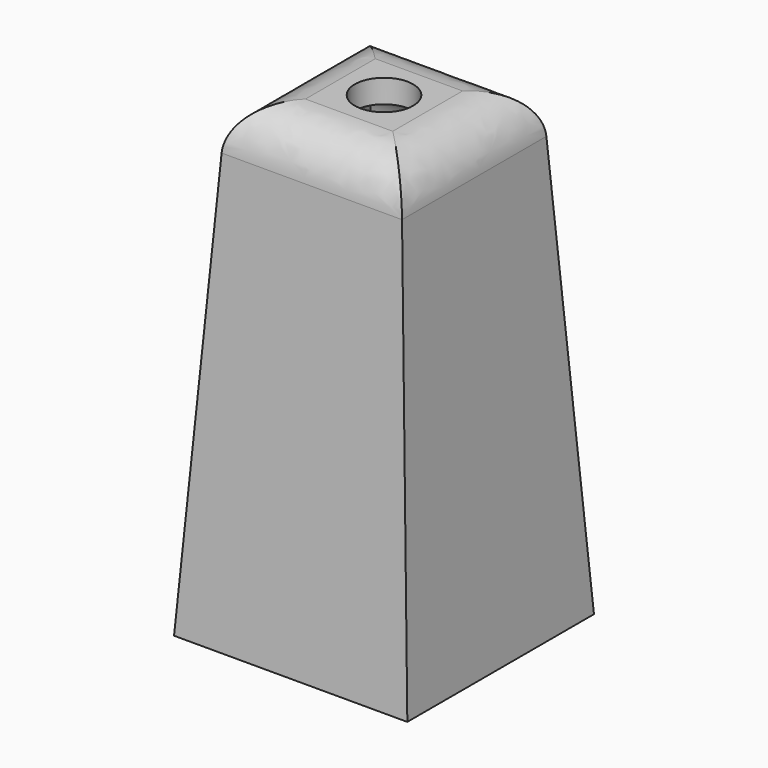
from build123d import *

# Parameters (mm, degrees)
F0_W     = 12.7
F0_H     = 12.7
F2_W     = 9.525
F2_H     = 9.525
F4_T     = -1.27
F5_R     = 1.5875
F6_DEPTH = 25.4
F7_R     = 2.54


with BuildPart() as f3:
    # F0 (on Top) → F3 section 0
    with BuildSketch(Plane.XY):
        with Locations((6.35, 6.35)):
            Rectangle(F0_W, F0_H)
    # F2 (on offset) → F3 section 1
    with BuildSketch(Plane.XY.offset(25.4)):
        with Locations((6.35, 6.35)):
            Rectangle(F2_W, F2_H)
    loft()

    # F4
    f4_openings = [f3.faces().sort_by_distance(p)[0] for p in [
        (6.35, 6.35, 0),
    ]]
    offset(amount=F4_T, openings=f4_openings)

    # F5 (on face) → F6 (cut)
    with BuildSketch(Plane.XY.offset(25.4)):
        with Locations((6.35, 6.35)):
            Circle(F5_R)
    extrude(amount=-F6_DEPTH, mode=Mode.SUBTRACT)

    # F7
    f7_edges = [f3.edges().sort_by_distance(p)[0] for p in [
        (6.35, 11.1125, 25.4),
        (11.1125, 6.35, 25.4),
        (6.35, 1.5875, 25.4),
        (1.5875, 6.35, 25.4),
        (9.919397, 6.35, 24.13),
        (6.35, 9.919397, 24.13),
        (2.780603, 6.35, 24.13),
        (6.35, 2.780603, 24.13),
    ]]
    fillet(f7_edges, radius=F7_R)


solid = f3.part
